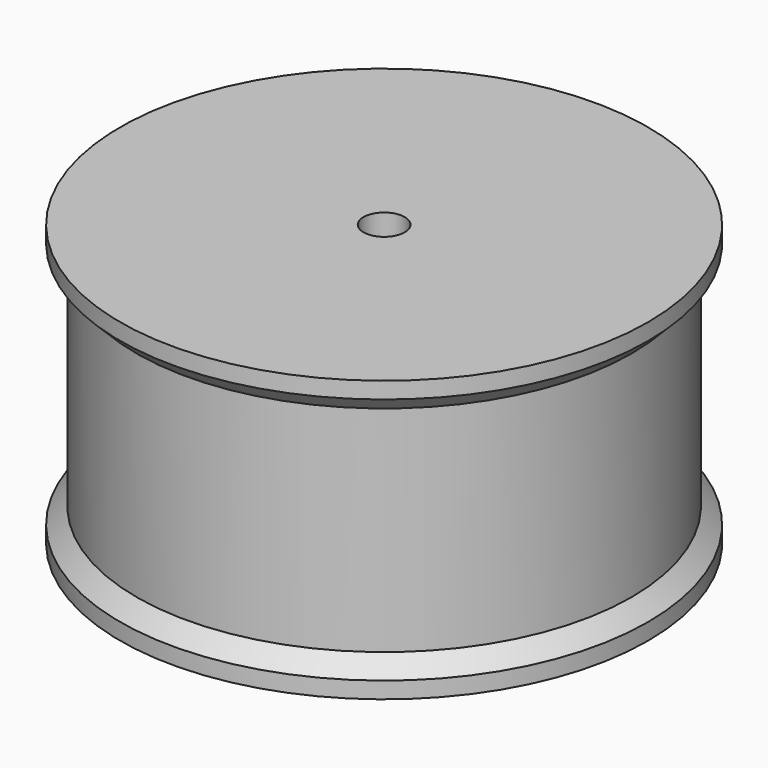
from build123d import *

# Parameters (mm, degrees)
F0_R      = 16
F1_DEPTH  = 2
F2_SIZE   = 1
F4_R      = 15
F5_DEPTH  = 13
F6_R      = 16
F7_DEPTH  = 1
F8_SIZE   = 0.99999
F9_DEPTH  = 1
F10_R     = 1.25
F11_DEPTH = 2.5
F12_D     = 2.5


# Not quite as in the source:
# - a fillet or chamfer is up to 0.001 mm smaller than in the source, because OpenCascade refuses the exact size


with BuildPart() as f1:
    # F0 (on Top) → F1 (new body)
    with BuildSketch(Plane.XY):
        Circle(F0_R)
    extrude(amount=F1_DEPTH)

    # F2
    f2_edges = [f1.edges().sort_by_distance(p)[0] for p in [
        (-16, 0, 2),
    ]]
    chamfer(f2_edges, length=F2_SIZE)

    # F4 (on face) → F5 (join)
    with BuildSketch(Plane.XY.offset(2)):
        Circle(F4_R)
    extrude(amount=F5_DEPTH)

    # F6 (on face) → F7 (join)
    with BuildSketch(Plane.XY.offset(15)):
        Circle(F6_R)
    extrude(amount=F7_DEPTH)

    # F8 (size 1 in the source; OpenCascade refuses exactly that, so slightly less here)
    f8_edges = [f1.edges().sort_by_distance(p)[0] for p in [
        (-16, 0, 15),
    ]]
    chamfer(f8_edges, length=F8_SIZE)

    # F9 (add): a face of the model
    f9_faces = [f1.faces().sort_by_distance(p)[0] for p in [
        (0, 0, 16),
    ]]
    extrude(f9_faces, amount=F9_DEPTH)

    # F10 (on face) → F11 (cut)
    with BuildSketch(Plane.XY):
        Circle(F10_R)
    extrude(amount=-F11_DEPTH, mode=Mode.SUBTRACT)

    # F12 (through all)
    with Locations(Plane(origin=(0, 0, 0), x_dir=(1, 0, 0), z_dir=(0, 0, -1))):
        with Locations((0, 0)):
            Hole(F12_D / 2)


solid = f1.part
